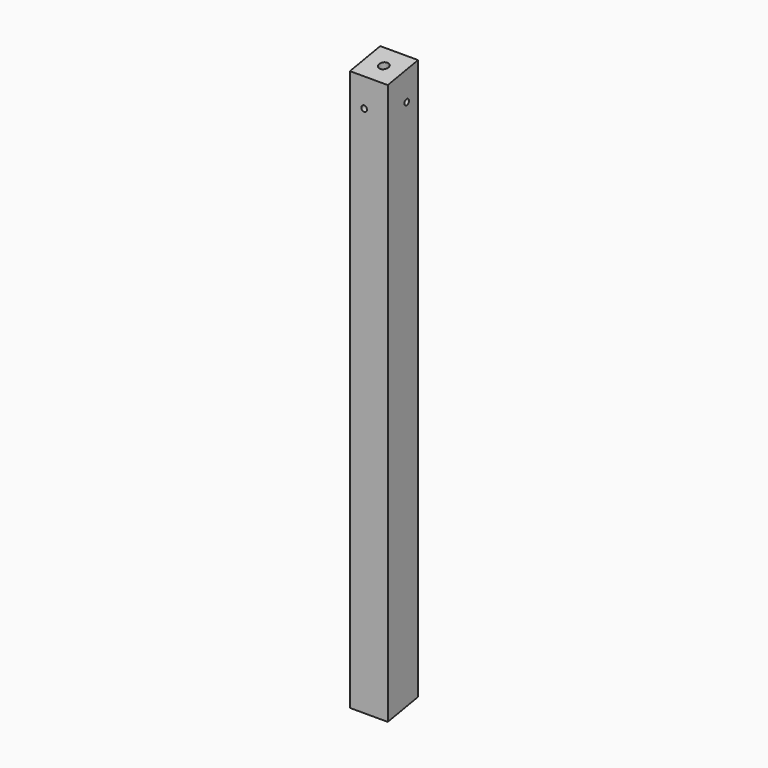
from build123d import *

# Parameters (mm, degrees)
F0_W        = 40
F0_H        = 40
F1_DEPTH    = 600
F3_T1_DEPTH = 247.8831037137
F4_R        = 3
F6_DEPTH    = 12
F5_R        = 3
F7_DEPTH    = 12
F8_R        = 5
F9_DEPTH    = 12


# Not quite as in the source:
# - a fillet or chamfer that OpenCascade refuses, or shapes differently, is made with other operations: its cross-section is extruded or revolved along the edge and cut away or added
# - a feature of the source that left no trace in its solid (it failed there, or was rolled back) is left out


with BuildPart() as f1:
    # F0 (on Top) → F1 (new body)
    with BuildSketch(Plane.XY):
        with Locations((20, 20)):
            Rectangle(F0_W, F0_H)
    extrude(amount=F1_DEPTH)

    # F3: chamfer of 40 x 7.0530792283 on 2 edges, made by hand

    # F3_s2 → F3_t1 (cut)
    with BuildSketch(Plane.YZ.offset(-103.9415518568)):
        Polygon((40, 7.0530792283), (0, 0), (40, 0), align=None)
        Polygon((0, 592.9469207717), (40, 600), (0, 600), align=None)
    extrude(amount=F3_T1_DEPTH, mode=Mode.SUBTRACT)

    # F4 (on face) → F6 (cut)
    with BuildSketch(Plane.XZ):
        with Locations((15, 562.9469207717)):
            Circle(F4_R)
    extrude(amount=-F6_DEPTH, mode=Mode.SUBTRACT)

    # F5 (on face) → F7 (cut)
    with BuildSketch(Plane.YZ.offset(40)):
        with Locations((25, 566.8922969328)):
            Circle(F5_R)
    extrude(amount=-F7_DEPTH, mode=Mode.SUBTRACT)

    # F8 (on face) → F9 (cut)
    with BuildSketch(Plane(origin=(0, -101.3998954134, 575.0673833693), x_dir=(1, 0, 0), z_dir=(0, -0.1736481777, 0.984807753))):
        with Locations((20.0023799473, 122.9641521036)):
            Circle(F8_R)
    extrude(amount=-F9_DEPTH, mode=Mode.SUBTRACT)


solid = f1.part
